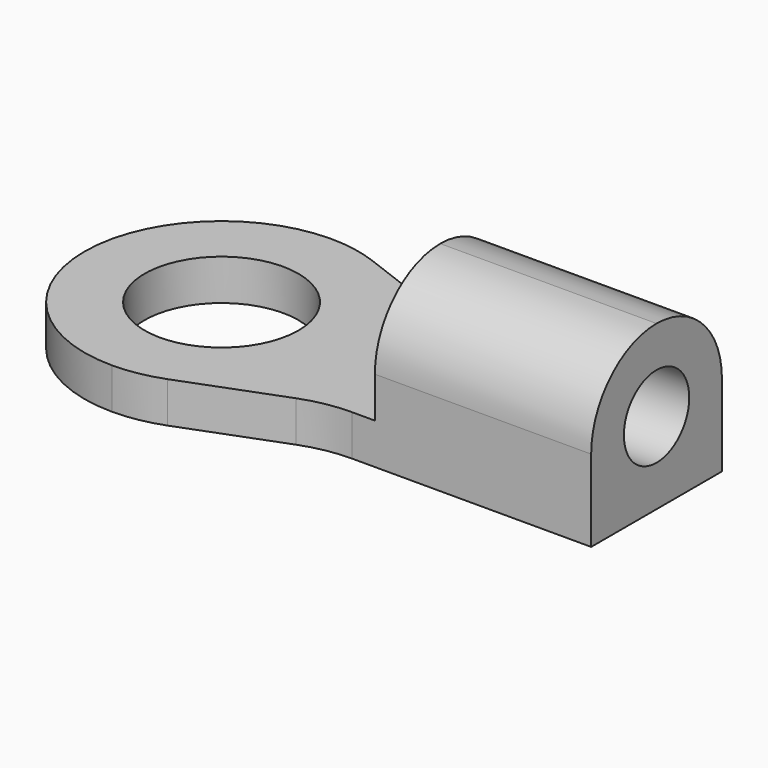
from build123d import *

# Parameters (mm, degrees)
F0_R     = 1.6
F1_DEPTH = 0.85
F2_W     = 4.5
F2_H     = 3.4
F3_DEPTH = 2.55
F4_R     = 1.69999
F5_R     = 0.85
F6_DEPTH = 25


# Not quite as in the source:
# - a fillet or chamfer is up to 0.001 mm smaller than in the source, because OpenCascade refuses the exact size


with BuildPart() as f1:
    # F0 (on Top) → F1 (new body)
    with BuildSketch(Plane.XY):
        with BuildLine():
            Line((6.9231632929, 1.15), (11.9, 1.15))
            Line((11.9, 1.15), (11.9, 4.55))
            Line((11.9, 4.55), (6.9231632929, 4.55))
            ThreePointArc((6.9231632929, 4.55), (6.408597702, 4.5968370984), (5.9109449246, 4.7358089455))
            Line((5.9109449246, 4.7358089455), (3.8622183683, 5.5141910545))
            ThreePointArc((3.8622183683, 5.5141910545), (3.3645655909, 5.6531629016), (2.85, 5.7))
            ThreePointArc((2.85, 5.7), (0.8347456736, 4.8652543264), (0, 2.85))
            ThreePointArc((0, 2.85), (0.8347456736, 0.8347456736), (2.85, 0))
            ThreePointArc((2.85, 0), (3.3645655909, 0.0468370984), (3.8622183683, 0.1858089455))
            Line((3.8622183683, 0.1858089455), (5.9109449246, 0.9641910545))
            ThreePointArc((5.9109449246, 0.9641910545), (6.408597702, 1.1031629016), (6.9231632929, 1.15))
        make_face()
        with Locations((2.85, 2.85)):
            Circle(F0_R, mode=Mode.SUBTRACT)
    extrude(amount=F1_DEPTH)

    # F2 (on face) → F3 (join)
    with BuildSketch(Plane.XY.offset(0.85)):
        with Locations((9.65, 2.85)):
            Rectangle(F2_W, F2_H)
    extrude(amount=F3_DEPTH)

    # F4 (radius 1.7 in the source; OpenCascade refuses exactly that, so slightly less here)
    f4_edges = [f1.edges().sort_by_distance(p)[0] for p in [
        (9.65, 4.55, 3.4),
        (9.65, 1.15, 3.4),
    ]]
    fillet(f4_edges, radius=F4_R)

    # F5 (on face) → F6 (cut)
    with BuildSketch(Plane.YZ.offset(11.9)):
        with Locations((2.85, 1.7)):
            Circle(F5_R)
    extrude(amount=-F6_DEPTH, mode=Mode.SUBTRACT)


solid = f1.part
